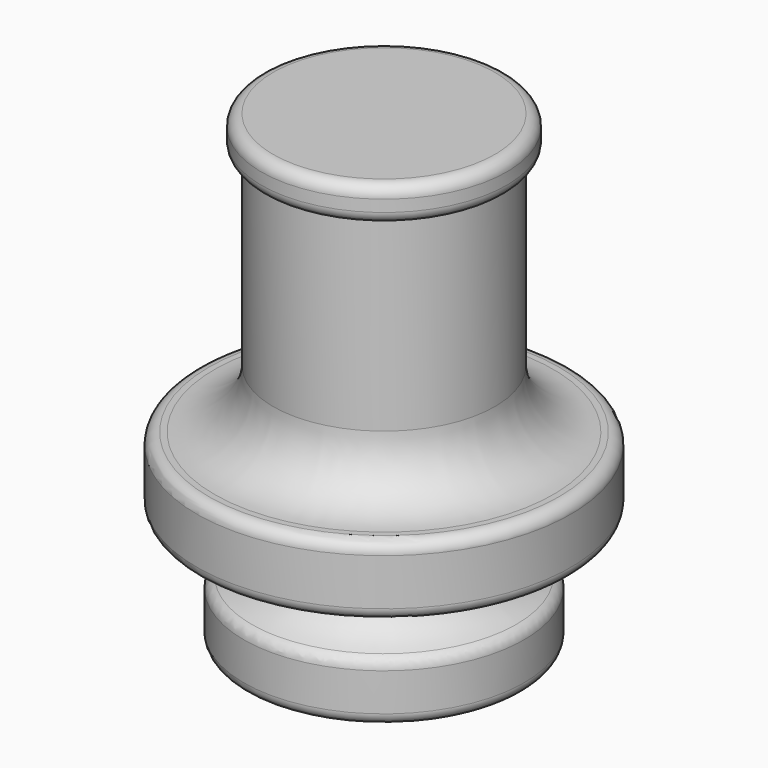
from build123d import *

# Parameters (mm, degrees)
F2_R = 0.99999
F4_R = 1


# Not quite as in the source:
# - a fillet or chamfer that OpenCascade refuses, or shapes differently, is made with other operations: its cross-section is extruded or revolved along the edge and cut away or added
# - a fillet or chamfer is up to 0.001 mm smaller than in the source, because OpenCascade refuses the exact size


with BuildPart() as f1:
    # F0 (on Right) → F1 (revolve)
    with BuildSketch(Plane.YZ):
        Polygon((0, -10), (0, 0), (-8, 0), (-8, -5), (-12, -5), (-12, -10), align=None)
        Polygon((-8, 0), (0, 0), (0, 30), (-10.5, 30), (-10.5, 27), (-9.5, 27), (-9.5, 6), (-16, 6), (-16, 0), align=None)
    revolve(axis=Axis((0, 0, 25.4025327901), (0, 0, 1)))

    # F2 (radius 1 in the source; OpenCascade refuses exactly that, so slightly less here)
    f2_edges = [f1.edges().sort_by_distance(p)[0] for p in [
        (0, 10.5, 30),
        (0, 10.5, 27),
    ]]
    fillet(f2_edges, radius=F2_R)

    # F3: fillet of radius 5 on 2 edges, made by hand

    # F3_s1 → F3_t2 (revolve)
    with BuildSketch(Plane.YZ):
        with BuildLine():
            ThreePointArc((-9.5, 11), (-10.9644660941, 7.4644660941), (-14.5, 6))
            Line((-14.5, 6), (-9.5, 6))
            Line((-9.5, 6), (-9.5, 11))
        make_face()
    revolve(axis=Axis((0, 0, 6), (0, 0, 1)))

    # F3_s3 → F3_t4 (revolve)
    with BuildSketch(Plane.YZ):
        with BuildLine():
            ThreePointArc((-8, -0.1010205144), (-9.1270166538, -3.2632981746), (-12, -5))
            Line((-12, -5), (-8, -5))
            Line((-8, -5), (-8, -0.1010205144))
        make_face()
    revolve(axis=Axis((0, 0, -5), (0, 0, 1)))

    # F4
    f4_edges = [f1.edges().sort_by_distance(p)[0] for p in [
        (0, 16, 6),
        (0, 16, 0),
        (0, 12, -5),
        (0, 12, -10),
    ]]
    fillet(f4_edges, radius=F4_R)


solid = f1.part
